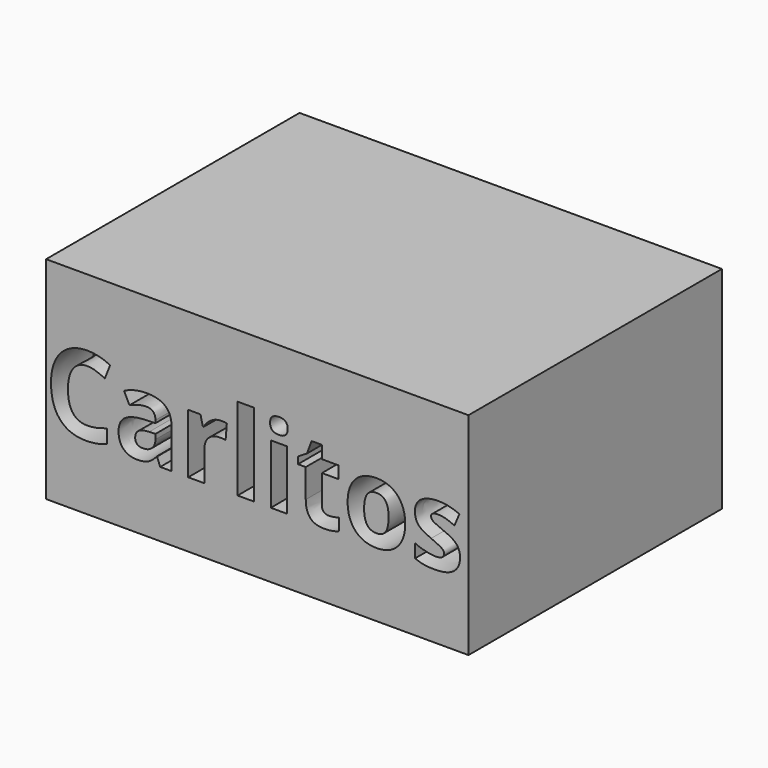
from build123d import *

# Parameters (mm, degrees)
F0_W         = 76.2
F0_H         = 50.8
F1_DEPTH     = 101.6
F2_TEXT_SIZE = 26.1665995976
F3_DEPTH     = 12.7


# Not quite as in the source:
# - Text() gives the source's letters only with a copy of the font that has no kerning and outlines rounded to 1/6400 em; it was checked with that copy


with BuildPart() as f1:
    # F0 (on Right) → F1 (new body)
    with BuildSketch(Plane.YZ):
        with Locations((-87.3882067442, -91.6964613557)):
            Rectangle(F0_W, F0_H)
    extrude(amount=F1_DEPTH)

    # F2 (on face) → F3 (cut)
    with BuildSketch(Plane.XZ.offset(125.4882067442)):
        with Locations((-0.3375909492, -101.3610564507)):
            Text('Carlitos', F2_TEXT_SIZE, font='Open Sans', font_style=FontStyle.BOLD, text_align=(TextAlign.LEFT, TextAlign.BOTTOM))
    extrude(amount=-F3_DEPTH, mode=Mode.SUBTRACT)


solid = f1.part
